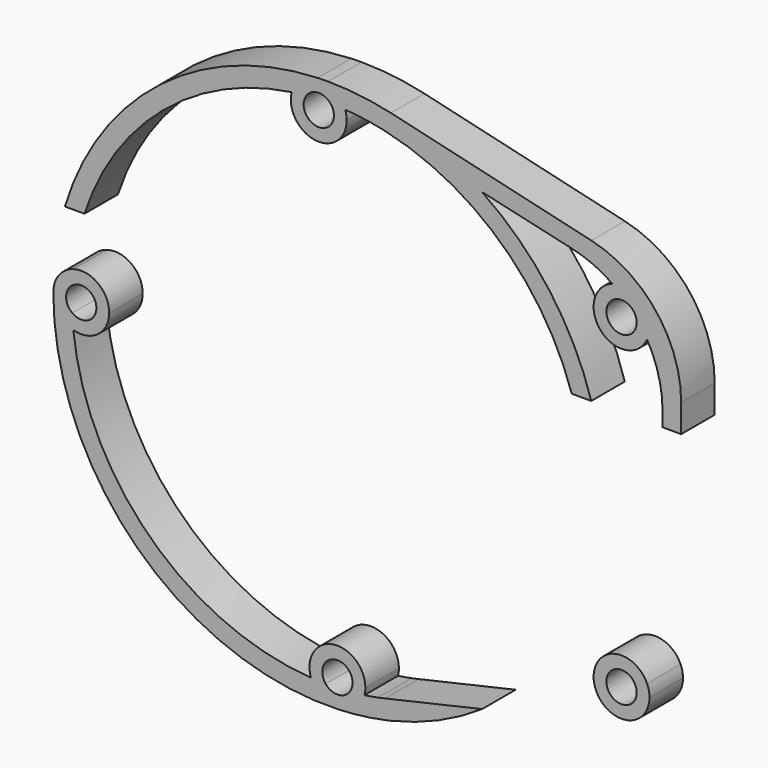
from build123d import *

# Parameters (mm, degrees)
F1_DEPTH = 9


# Not quite as in the source:
# - a feature names something its author has since deleted; it is built from what else it names


with BuildPart() as f1:
    # F0 (on Front) → F1 (new body)
    with BuildSketch(Plane.XZ):
        with BuildLine():
            ThreePointArc((2.2264151739, -58.9579771996), (7.3156733339, -58.544691678), (12.3501399093, -57.6929288927))
            ThreePointArc((12.3501399093, -57.6929288927), (12.7483225231, -57.6062520292), (13.1458969739, -57.51682704))
            ThreePointArc((13.1458969739, -57.51682704), (13.3201678722, -57.4767181375), (13.4943164015, -57.4360812108))
            ThreePointArc((13.4943164015, -57.4360812108), (23.6747774831, -54.0416960423), (33.0719942338, -48.8594228108))
            Line((33.0719942338, -48.8594228108), (12.2547311497, -53.617362528))
            ThreePointArc((12.2547311497, -53.6173625279), (11.4908249672, -53.7862523474), (10.724593739, -53.9442590934))
            ThreePointArc((10.724593739, -53.9442590934), (9.2729705564, -54.2126555064), (7.8146670139, -54.4419964684))
            ThreePointArc((7.8146670139, -54.4419964684), (5.7712317605, -57.6289209346), (2.2264151739, -58.9579771996))
        make_face()
        with BuildLine():
            ThreePointArc((-59, 0), (-40.9245739425, -42.499167611), (2.2264151739, -58.9579771996))
            ThreePointArc((2.2264151739, -58.9579771996), (-1.4085405992, -57.9000488994), (-3.6865075266, -54.8763123967))
            ThreePointArc((-3.6865075266, -54.8763123967), (-38.1500265832, -39.6178680862), (-54.6981132075, -5.75468605))
            ThreePointArc((-54.6981132075, -5.75468605), (-57.8056570438, -3.5924449025), (-59, 0))
        make_face()
        with BuildLine():
            ThreePointArc((-3.6865075266, -54.8763123967), (-1.4085405992, -57.9000488994), (2.2264151739, -58.9579771996))
            ThreePointArc((2.2264151739, -58.9579771996), (5.7712317605, -57.6289209346), (7.8146670139, -54.4419964684))
            ThreePointArc((7.8146670139, -54.4419964684), (6.2499884856, -54.643733803), (4.6801675765, -54.8005112335))
            ThreePointArc((4.6801675765, -54.8005112335), (2.1395152245, -56.2092547885), (-0.5126102579, -55.023631238))
            ThreePointArc((-0.5126102579, -55.023631238), (-0.523287524, -55.0105475784), (-0.5338966616, -54.9974086149))
            ThreePointArc((-0.5338966616, -54.9974086149), (-2.11107057, -54.9594703491), (-3.6865075266, -54.8763123967))
        make_face()
        with BuildLine():
            ThreePointArc((-54.6981132075, 5.75468605), (-57.8056570438, 3.5924449025), (-59, 0))
            ThreePointArc((-59, 0), (-57.8056570438, -3.5924449025), (-54.6981132075, -5.75468605))
            ThreePointArc((-54.6981132075, -5.75468605), (-54.8406623818, -4.1835092356), (-54.9380896226, -2.6088903033))
            ThreePointArc((-54.9380896226, -2.6088903033), (-56.25, 0), (-54.9380896226, 2.6088903033))
            ThreePointArc((-54.9380896226, 2.6088903033), (-54.8406623818, 4.1835092356), (-54.6981132075, 5.75468605))
        make_face()
        with BuildLine():
            ThreePointArc((8, -52.9622507075), (1.0302178491, -47.0411424852), (-3.6865075266, -54.8763123967))
            ThreePointArc((-3.6865075266, -54.8763123967), (-2.11107057, -54.9594703491), (-0.5338966616, -54.9974086149))
            ThreePointArc((-0.5338966616, -54.9974086149), (0.9212655911, -49.8964992376), (5.25, -52.9622507075))
            ThreePointArc((5.25, -52.9622507075), (5.1042748448, -53.9245280522), (4.6801675765, -54.8005112335))
            ThreePointArc((4.6801675765, -54.8005112335), (6.2499884856, -54.643733803), (7.8146670139, -54.4419964684))
            ThreePointArc((7.8146670139, -54.4419964684), (7.953486461, -53.7079040841), (8, -52.9622507075))
        make_face()
        with BuildLine():
            ThreePointArc((-47, 0), (-49.4075550975, 4.8056570438), (-54.6981132075, 5.75468605))
            ThreePointArc((-54.6981132075, 5.75468605), (-54.8406623818, 4.1835092356), (-54.9380896226, 2.6088903033))
            ThreePointArc((-54.9380896226, 2.6088903033), (-51.5399128919, 2.9035574106), (-49.75, 0))
            ThreePointArc((-49.75, 0), (-51.5399128919, -2.9035574106), (-54.9380896226, -2.6088903033))
            ThreePointArc((-54.9380896226, -2.6088903033), (-54.8406623818, -4.1835092356), (-54.6981132075, -5.75468605))
            ThreePointArc((-54.6981132075, -5.75468605), (-49.4075550975, -4.8056570438), (-47, 0))
        make_face()
    extrude(amount=F1_DEPTH)


with BuildPart() as f1b:
    # F0 (on Front) → F1, piece 2 (new body)
    with BuildSketch(Plane.XZ):
        with BuildLine():
            ThreePointArc((-2.2264152072, 58.9579771984), (-36.0875389034, 46.6764344814), (-56.4983880681, 16.9980041683))
            Line((-56.4983880681, 16.9980041683), (-52.3074359369, 16.9980041683))
            ThreePointArc((-52.3074359369, 16.9980041683), (-35.4144032231, 42.0811126795), (-7.8146670139, 54.4419964684))
            ThreePointArc((-7.8146670139, 54.4419964684), (-5.7712317735, 57.6289209241), (-2.2264152072, 58.9579771984))
        make_face()
        with BuildLine():
            ThreePointArc((0, 59), (-1.1134058773, 58.9894933641), (-2.2264152072, 58.9579771984))
            ThreePointArc((-2.2264152072, 58.9579771984), (1.4085405854, 57.9000489088), (3.6865075266, 54.8763123967))
            ThreePointArc((3.6865075266, 54.8763123967), (7.5029468578, 54.4858310797), (11.2828817239, 53.8302571051))
            Line((11.2828817239, 53.8302571051), (11.6555883217, 53.7543010605))
            Line((11.6555883217, 53.7543010605), (12.2546497214, 53.617381139))
            Line((12.2546497214, 53.617381139), (33.0719942338, 48.8594228108))
            ThreePointArc((33.0719942338, 48.8594228108), (23.6747775211, 54.0416960256), (13.4943164822, 57.4360811919))
            ThreePointArc((13.4943164822, 57.4360811919), (6.7923195479, 58.6077161742), (0, 59))
        make_face()
        with BuildLine():
            ThreePointArc((3.6865075266, 54.8763123967), (1.4085405854, 57.9000489088), (-2.2264152072, 58.9579771984))
            ThreePointArc((-2.2264152072, 58.9579771984), (-5.7712317735, 57.6289209241), (-7.8146670139, 54.4419964684))
            ThreePointArc((-7.8146670139, 54.4419964684), (-6.2499884856, 54.643733803), (-4.6801675765, 54.8005112335))
            ThreePointArc((-4.6801675765, 54.8005112335), (-2.1226415094, 56.2099358924), (0.5338966616, 54.9974086149))
            ThreePointArc((0.5338966616, 54.9974086149), (2.11107057, 54.9594703491), (3.6865075266, 54.8763123967))
        make_face()
        with BuildLine():
            Line((52.3074359369, 16.9980041683), (56.4983880681, 16.9980041683))
            ThreePointArc((56.4983880681, 16.9980041683), (47.5342071135, 34.9499521329), (33.0719942338, 48.8594228108))
            Line((33.0719942338, 48.8594228108), (12.2546497214, 53.617381139))
            ThreePointArc((12.2546497214, 53.617381139), (37.1121330372, 40.591742774), (52.3074359369, 16.9980041683))
        make_face()
        with BuildLine():
            ThreePointArc((4, 52.9622507075), (3.9211082223, 53.9320328584), (3.6865075266, 54.8763123967))
            ThreePointArc((3.6865075266, 54.8763123967), (2.11107057, 54.9594703491), (0.5338966616, 54.9974086149))
            ThreePointArc((0.5338966616, 54.9974086149), (1.0657514699, 54.0409851163), (1.25, 52.9622507075))
            ThreePointArc((1.25, 52.9622507075), (-2.9622773447, 49.8579758627), (-4.6801675765, 54.8005112335))
            ThreePointArc((-4.6801675765, 54.8005112335), (-6.2499884856, 54.643733803), (-7.8146670139, 54.4419964684))
            ThreePointArc((-7.8146670139, 54.4419964684), (-2.7456533767, 47.0087642464), (4, 52.9622507075))
        make_face()
        with BuildLine():
            ThreePointArc((13.4943164822, 57.4360811919), (23.6747775211, 54.0416960256), (33.0719942338, 48.8594228108))
            Line((33.0719942338, 48.8594228108), (52.3755635072, 44.4474490293))
            ThreePointArc((52.3755635072, 44.4474490293), (56.8873510456, 42.9527914166), (61.0347281001, 40.631263528))
            ThreePointArc((61.0347281001, 40.631263528), (66.4791068251, 39.8505853625), (69, 34.9622507075))
            ThreePointArc((69, 34.9622507075), (68.8695285228, 33.7178090977), (68.48378836, 32.5274888663))
            ThreePointArc((68.48378836, 32.5274888663), (70.9606299497, 26.5193970545), (71.8052681793, 20.0759121479))
            Line((71.8052681793, 20.0759121479), (71.8052681793, 16.9980041683))
            Line((71.8052681793, 16.9980041683), (75.8052681793, 16.9980041683))
            Line((75.8052681793, 16.9980041683), (75.8052681793, 22.9893407228))
            ThreePointArc((75.8052681793, 22.9893407228), (70.4005260997, 38.5143485177), (56.5231988167, 47.3266632794))
            Line((56.5231988167, 47.3266632794), (13.4943164822, 57.4360811919))
        make_face()
        with BuildLine():
            ThreePointArc((64.2884750409, 37.9459283155), (62.7183466029, 39.3573523193), (61.0347281001, 40.631263528))
            ThreePointArc((61.0347281001, 40.631263528), (58.5826727015, 30.901804976), (68.48378836, 32.5274888663))
            ThreePointArc((68.48378836, 32.5274888663), (67.3558810778, 34.3122146697), (66.0814094211, 35.9954089623))
            ThreePointArc((66.0814094211, 35.9954089623), (66.2075754565, 35.4856622957), (66.25, 34.9622507075))
            ThreePointArc((66.25, 34.9622507075), (60.2843008374, 33.1768997452), (64.2884750409, 37.9459283155))
        make_face()
        with BuildLine():
            ThreePointArc((69, 34.9622507075), (66.4791068251, 39.8505853625), (61.0347281001, 40.631263528))
            ThreePointArc((61.0347281001, 40.631263528), (62.7183466029, 39.3573523193), (64.2884750409, 37.9459283155))
            ThreePointArc((64.2884750409, 37.9459283155), (65.3927189533, 37.161658812), (66.0814094211, 35.9954089623))
            ThreePointArc((66.0814094211, 35.9954089623), (67.3558810778, 34.3122146697), (68.48378836, 32.5274888663))
            ThreePointArc((68.48378836, 32.5274888663), (68.8695285228, 33.7178090977), (69, 34.9622507075))
        make_face()
    extrude(amount=F1_DEPTH)


with BuildPart() as f1c:
    # F0 (on Front) → F1, piece 3 (new body)
    with BuildSketch(Plane.XZ):
        with BuildLine():
            ThreePointArc((64.2884750409, -37.9459283155), (62.7183466029, -39.3573523193), (61.0347281001, -40.631263528))
            ThreePointArc((61.0347281001, -40.631263528), (66.4791068251, -39.8505853625), (69, -34.9622507075))
            ThreePointArc((69, -34.9622507075), (68.8695285228, -33.7178090977), (68.48378836, -32.5274888663))
            ThreePointArc((68.48378836, -32.5274888663), (67.3558810778, -34.3122146697), (66.0814094211, -35.9954089623))
            ThreePointArc((66.0814094211, -35.9954089623), (65.3927189533, -37.161658812), (64.2884750409, -37.9459283155))
        make_face()
        with BuildLine():
            ThreePointArc((68.48378836, -32.5274888663), (58.5826727015, -30.901804976), (61.0347281001, -40.631263528))
            ThreePointArc((61.0347281001, -40.631263528), (62.7183466029, -39.3573523193), (64.2884750409, -37.9459283155))
            ThreePointArc((64.2884750409, -37.9459283155), (60.2843008374, -33.1768997452), (66.25, -34.9622507075))
            ThreePointArc((66.25, -34.9622507075), (66.2075754565, -35.4856622957), (66.0814094211, -35.9954089623))
            ThreePointArc((66.0814094211, -35.9954089623), (67.3558810778, -34.3122146697), (68.48378836, -32.5274888663))
        make_face()
    extrude(amount=F1_DEPTH)


solid = Compound([f1.part, f1b.part, f1c.part])
